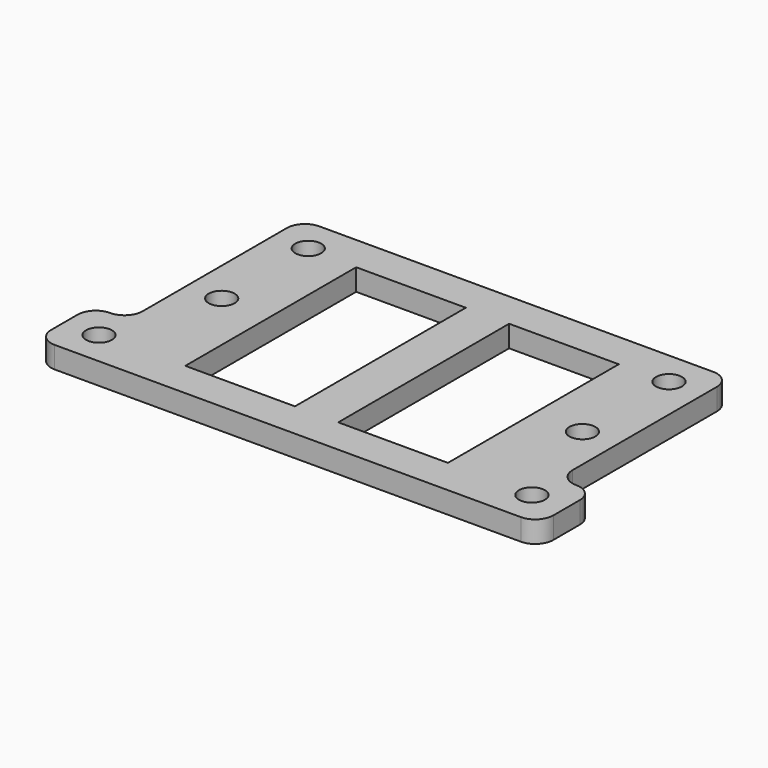
from build123d import *

# Parameters (mm, degrees)
F0_R     = 1.8
F1_DEPTH = 3
F2_R     = 2.49999
F3_W     = 15.2
F3_H     = 29.6
F4_DEPTH = 3


# Not quite as in the source:
# - a fillet or chamfer is up to 0.001 mm smaller than in the source, because OpenCascade refuses the exact size


with BuildPart() as f1:
    # F0 (on Top) → F1 (new body)
    with BuildSketch(Plane.XY):
        Polygon((-34.8, 9.6), (-34.8, 0), (34.8, 0), (34.8, 9.6), (29.8, 9.6), (29.8, 39.6), (-29.8, 39.6), (-29.8, 9.6), align=None)
        with Locations((-30, 4.8)):
            Circle(F0_R, mode=Mode.SUBTRACT)
        with Locations((30, 4.8)):
            Circle(F0_R, mode=Mode.SUBTRACT)
        with Locations((-25, 19.8)):
            Circle(F0_R, mode=Mode.SUBTRACT)
        with Locations((-25, 34.8)):
            Circle(F0_R, mode=Mode.SUBTRACT)
        with Locations((25, 19.8)):
            Circle(F0_R, mode=Mode.SUBTRACT)
        with Locations((25, 34.8)):
            Circle(F0_R, mode=Mode.SUBTRACT)
    extrude(amount=F1_DEPTH)

    # F2 (radius 2.5 in the source; OpenCascade refuses exactly that, so slightly less here)
    f2_edges = [f1.edges().sort_by_distance(p)[0] for p in [
        (-34.8, 0, 1.5),
        (-34.8, 9.6, 1.5),
        (-29.8, 9.6, 1.5),
        (34.8, 0, 1.5),
        (29.8, 9.6, 1.5),
        (34.8, 9.6, 1.5),
        (29.8, 39.6, 1.5),
        (-29.8, 39.6, 1.5),
    ]]
    fillet(f2_edges, radius=F2_R)

    # F3 (on face) → F4 (cut, through all)
    with BuildSketch(Plane(origin=(0, 0, 0), x_dir=(1, 0, 0), z_dir=(0, 0, -1))):
        with Locations((10.6, -19.8)):
            Rectangle(F3_W, F3_H)
        with Locations((-10.6, -19.8)):
            Rectangle(F3_W, F3_H)
    extrude(amount=-F4_DEPTH, mode=Mode.SUBTRACT)


solid = f1.part
